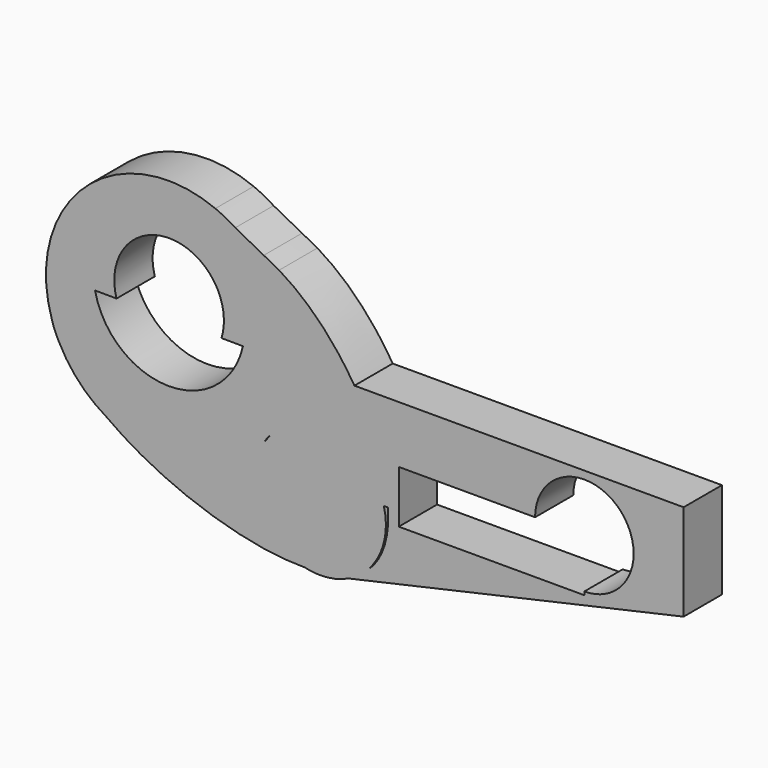
from build123d import *

# Parameters (mm, degrees)
F1_DEPTH = 25.4


with BuildPart() as f1:
    # F0 (on Front) → F1 (new body)
    with BuildSketch(Plane.XZ):
        with BuildLine():
            ThreePointArc((-23.4881200852, 9.1129863922), (-25.7569087098, 4.6952436795), (-27.3750988376, 0))
            ThreePointArc((-27.3750988376, 0), (-23.4523587377, -26.5236540337), (-1.822285639, -42.3676450379))
            add(Edge.make_bspline(
                [(31.6214489009, -32.408137431), (24.0381488742, -39.1257279454), (12.1793845571, -42.1949100042), (-1.822285639, -42.3676450379)],
                knots=[0.3305657958, 0.3305657958, 0.3305657958, 0.3305657958, 0.4117411776, 0.4117411776, 0.4117411776, 0.4117411776], degree=3))
            ThreePointArc((31.6214489009, -32.408137431), (39.9732334064, -17.2802023076), (40.0097537836, 0))
            Line((40.0097537836, 0), (24.3855283995, 0))
            Line((24.3855283995, 0), (24.3855283995, 20.8383404807))
            ThreePointArc((24.3855283995, 20.8383404808), (0.9049170427, 25.4619632407), (-20.0263610495, 13.8602998023))
            ThreePointArc((-20.0263610495, 13.8602998023), (-21.7035792641, 11.4475130703), (-23.4881200852, 9.1129863922))
        make_face()
        with BuildLine():
            ThreePointArc((-1.822285639, -42.3676450379), (-23.4523587377, -26.5236540337), (-27.3750988376, 0))
            ThreePointArc((-27.3750988376, 0), (-25.7569087098, 4.6952436795), (-23.4881200852, 9.1129863922))
            ThreePointArc((-23.4881200852, 9.1129863922), (-62.2831037982, -14.1508466737), (-106.8623494937, -6.4731163171))
            add(Edge.make_bspline(
                [(-1.822285639, -42.3676450379), (-34.1627739251, -42.7666213928), (-77.9356396487, -27.7130872373), (-106.8623494937, -6.4731163171)],
                knots=[0.4117411776, 0.4117411776, 0.4117411776, 0.4117411776, 0.5992367726, 0.5992367726, 0.5992367726, 0.5992367726], degree=3))
        make_face()
        with BuildLine():
            add(Edge.make_bspline(
                [(31.6214489009, -32.408137431), (24.0381488742, -39.1257279454), (12.1793845571, -42.1949100042), (-1.822285639, -42.3676450379)],
                knots=[0.3305657958, 0.3305657958, 0.3305657958, 0.3305657958, 0.4117411776, 0.4117411776, 0.4117411776, 0.4117411776], degree=3))
            ThreePointArc((-1.822285639, -42.3676450379), (2.2189423584, -43.0915267187), (6.317327473, -43.3339475664))
            Line((6.317327473, -43.3339475664), (21.2019422511, -39.9863561607))
            ThreePointArc((21.2019422511, -39.9863561607), (26.7658232425, -36.6841469116), (31.6214489009, -32.408137431))
        make_face()
        with BuildLine():
            ThreePointArc((-106.8623494937, -6.4731163171), (-62.2831037982, -14.1508466737), (-23.4881200852, 9.1129863922))
            ThreePointArc((-23.4881200852, 9.1129863922), (-21.8574061869, 11.5596842489), (-20.0263610495, 13.8602998023))
            ThreePointArc((-20.0263610495, 13.8602998023), (-11.9815447312, 31.0090830109), (-9.2218346427, 49.7489825666))
            ThreePointArc((-9.2218346427, 49.7489825666), (-15.373040222, 77.3515736193), (-32.6625531747, 99.7304275837))
            add(Edge.make_bspline(
                [(-136.0971185339, 29.794675775), (-147.1795152867, 70.6622045283), (-83.4949169934, 115.3318185014), (-32.6625531747, 99.7304275837)],
                knots=[0.6952883419, 0.6952883419, 0.6952883419, 0.6952883419, 1, 1, 1, 1], degree=3))
            ThreePointArc((-136.0971185339, 29.794675775), (-134.3309912676, 24.9782257744), (-132.1905665466, 20.3160397911))
            add(Edge.make_bspline(
                [(-106.8623494937, -6.4731163171), (-118.0127633165, 1.7142809574), (-126.9572157407, 10.8209088266), (-132.1905665466, 20.3160397911)],
                knots=[0.5992367726, 0.5992367726, 0.5992367726, 0.5992367726, 0.6715109264, 0.6715109264, 0.6715109264, 0.6715109264], degree=3))
        make_face()
        with BuildLine():
            ThreePointArc((-34.7453205512, 50.2754222832), (-74.1782043044, 18.8325014661), (-113.1855020537, 50.8018666913))
            Line((-113.1855020537, 50.8018666913), (-101.7999106632, 50.7254532919))
            ThreePointArc((-101.7999106632, 50.7254532918), (-78.0602804594, 87.7213526899), (-44.8327322387, 58.9429466583))
            ThreePointArc((-44.8327322387, 58.9429466583), (-45.1591089284, 54.5986268514), (-46.1309119417, 50.3518356826))
            Line((-46.1309119417, 50.3518356826), (-34.7453205512, 50.2754222832))
        make_face(mode=Mode.SUBTRACT)
        with BuildLine():
            Line((21.2019422511, -39.9863561607), (6.317327473, -43.3339475664))
            ThreePointArc((6.317327473, -43.3339475664), (13.9455337712, -42.486726351), (21.2019422511, -39.9863561607))
        make_face()
        with BuildLine():
            add(Edge.make_bspline(
                [(42.2519440934, 0), (43.0667519502, -13.4532818738), (39.8786763522, -25.0935550451), (31.6214489009, -32.408137431)],
                knots=[0.2421763625, 0.2421763625, 0.2421763625, 0.2421763625, 0.3305657958, 0.3305657958, 0.3305657958, 0.3305657958], degree=3))
            ThreePointArc((31.6214489009, -32.408137431), (26.7658232425, -36.6841469116), (21.2019422511, -39.9863561607))
            Line((21.2019422511, -39.9863561607), (198.9958948854, 0))
            Line((198.9958948854, 0), (162.1864286042, 0))
            ThreePointArc((162.1864286042, 0), (154.7074790766, -3.9710732295), (146.3514873037, -5.3427547241))
            Line((146.3514873037, -5.3427547241), (146.3514873037, -7.1069937982))
            Line((146.3514873037, -7.1069937982), (47.9064245235, -7.1069937982))
            Line((47.9064245235, -7.1069937982), (47.9064245235, 0))
            Line((47.9064245235, 0), (42.2519440934, 0))
        make_face()
        with BuildLine():
            ThreePointArc((-132.1905665466, 20.3160397911), (-121.4653525437, 5.0883042782), (-106.8623494937, -6.4731163171))
            add(Edge.make_bspline(
                [(-106.8623494937, -6.4731163171), (-118.0127633165, 1.7142809574), (-126.9572157407, 10.8209088266), (-132.1905665466, 20.3160397911)],
                knots=[0.5992367726, 0.5992367726, 0.5992367726, 0.5992367726, 0.6715109264, 0.6715109264, 0.6715109264, 0.6715109264], degree=3))
        make_face()
        with BuildLine():
            ThreePointArc((-9.2218346427, 49.7489825666), (-11.9815447312, 31.0090830109), (-20.0263610495, 13.8602998023))
            ThreePointArc((-20.0263610495, 13.8602998023), (0.9049170427, 25.4619632407), (24.3855283995, 20.8383404808))
            Line((24.3855283995, 20.8383404807), (24.3855283995, 51.0906824548))
            add(Edge.make_bspline(
                [(-15.5554291457, 92.0261433749), (0.3390335994, 82.5415688484), (14.2065732282, 67.591169523), (24.3855283995, 51.0906824548)],
                knots=[0.0353561549, 0.0353561549, 0.0353561549, 0.0353561549, 0.1378329831, 0.1378329831, 0.1378329831, 0.1378329831], degree=3))
            Line((-15.5554291457, 92.0261433749), (-23.7091819765, 96.3155100856))
            add(Edge.make_bspline(
                [(-32.6625531747, 99.7304275837), (-29.6292369493, 98.7994468334), (-26.6416857173, 97.653849539), (-23.7091819765, 96.3155100856)],
                knots=[0, 0, 0, 0, 0.0181830383, 0.0181830383, 0.0181830383, 0.0181830383], degree=3))
            ThreePointArc((-32.6625531747, 99.7304275837), (-15.373040222, 77.3515736193), (-9.2218346427, 49.7489825666))
        make_face()
        with BuildLine():
            Line((24.3855283995, 0), (40.0097537836, 0))
            ThreePointArc((40.0097537836, 0), (34.2162475505, 11.9326862666), (24.3855283995, 20.8383404808))
            Line((24.3855283995, 20.8383404807), (24.3855283995, 0))
        make_face()
        with BuildLine():
            ThreePointArc((24.3855283995, 20.8383404808), (34.2162475505, 11.9326862666), (40.0097537836, 0))
            Line((40.0097537836, 0), (42.2519440934, 0))
            add(Edge.make_bspline(
                [(24.3855283995, 51.0906824548), (34.7498868563, 34.2896493617), (41.2900666127, 15.8815465109), (42.2519440934, 0)],
                knots=[0.1378329831, 0.1378329831, 0.1378329831, 0.1378329831, 0.2421763625, 0.2421763625, 0.2421763625, 0.2421763625], degree=3))
            Line((24.3855283995, 51.0906824548), (24.3855283995, 20.8383404807))
        make_face()
        with BuildLine():
            add(Edge.make_bspline(
                [(24.3855283995, 51.0906824548), (34.7498868563, 34.2896493617), (41.2900666127, 15.8815465109), (42.2519440934, 0)],
                knots=[0.1378329831, 0.1378329831, 0.1378329831, 0.1378329831, 0.2421763625, 0.2421763625, 0.2421763625, 0.2421763625], degree=3))
            Line((42.2519440934, 0), (47.9064245235, 0))
            Line((47.9064245235, 0), (47.9064245235, 20.7945478899))
            Line((47.9064245235, 20.7945478899), (120.2141846897, 20.7945478899))
            ThreePointArc((120.2141846897, 20.7945478899), (146.3514873037, 46.931850504), (172.4887899177, 20.7945478899))
            ThreePointArc((172.4887899177, 20.7945478899), (169.7720043836, 9.1911877022), (162.1864286042, 0))
            Line((162.1864286042, 0), (198.9958948854, 0))
            Line((198.9958948854, 0), (198.9958948854, 51.0906824548))
            Line((198.9958948854, 51.0906824548), (24.3855283995, 51.0906824548))
        make_face()
        with BuildLine():
            add(Edge.make_bspline(
                [(-132.1905665466, 20.3160397911), (-133.9122824029, 23.4398352609), (-135.2323312991, 26.6056799314), (-136.0971185339, 29.794675775)],
                knots=[0.6715109264, 0.6715109264, 0.6715109264, 0.6715109264, 0.6952883419, 0.6952883419, 0.6952883419, 0.6952883419], degree=3))
            ThreePointArc((-132.1905665466, 20.3160397911), (-134.3309912676, 24.9782257744), (-136.0971185339, 29.794675775))
        make_face()
        with BuildLine():
            ThreePointArc((-49.373536191, 109.8165112697), (-118.3123179762, 97.5246309308), (-136.0971185339, 29.794675775))
            add(Edge.make_bspline(
                [(-136.0971185339, 29.794675775), (-147.1795152867, 70.6622045283), (-83.4949169934, 115.3318185014), (-32.6625531747, 99.7304275837)],
                knots=[0.6952883419, 0.6952883419, 0.6952883419, 0.6952883419, 1, 1, 1, 1], degree=3))
            ThreePointArc((-32.6625531747, 99.7304275837), (-35.6692605933, 102.0849992123), (-38.8090434498, 104.2589496877))
            Line((-38.8090434498, 104.2589496877), (-49.373536191, 109.8165112697))
        make_face()
        with BuildLine():
            ThreePointArc((-38.8090434498, 104.2589496877), (-35.6692605933, 102.0849992123), (-32.6625531747, 99.7304275837))
            add(Edge.make_bspline(
                [(-32.6625531747, 99.7304275837), (-29.6292369493, 98.7994468334), (-26.6416857173, 97.653849539), (-23.7091819765, 96.3155100856)],
                knots=[0, 0, 0, 0, 0.0181830383, 0.0181830383, 0.0181830383, 0.0181830383], degree=3))
            Line((-23.7091819765, 96.3155100856), (-38.8090434498, 104.2589496877))
        make_face()
        with BuildLine():
            Line((-23.7091819765, 96.3155100856), (-15.5554291457, 92.0261433749))
            add(Edge.make_bspline(
                [(-23.7091819765, 96.3155100856), (-20.9395552466, 95.0515046312), (-18.2190309331, 93.615572981), (-15.5554291457, 92.0261433749)],
                knots=[0.0181830383, 0.0181830383, 0.0181830383, 0.0181830383, 0.0353561549, 0.0353561549, 0.0353561549, 0.0353561549], degree=3))
        make_face()
        with BuildLine():
            ThreePointArc((-38.8090434498, 104.2589496877), (-43.9634537245, 107.2807369641), (-49.373536191, 109.8165112697))
            Line((-49.373536191, 109.8165112697), (-38.8090434498, 104.2589496877))
        make_face()
    extrude(amount=F1_DEPTH)


solid = f1.part
